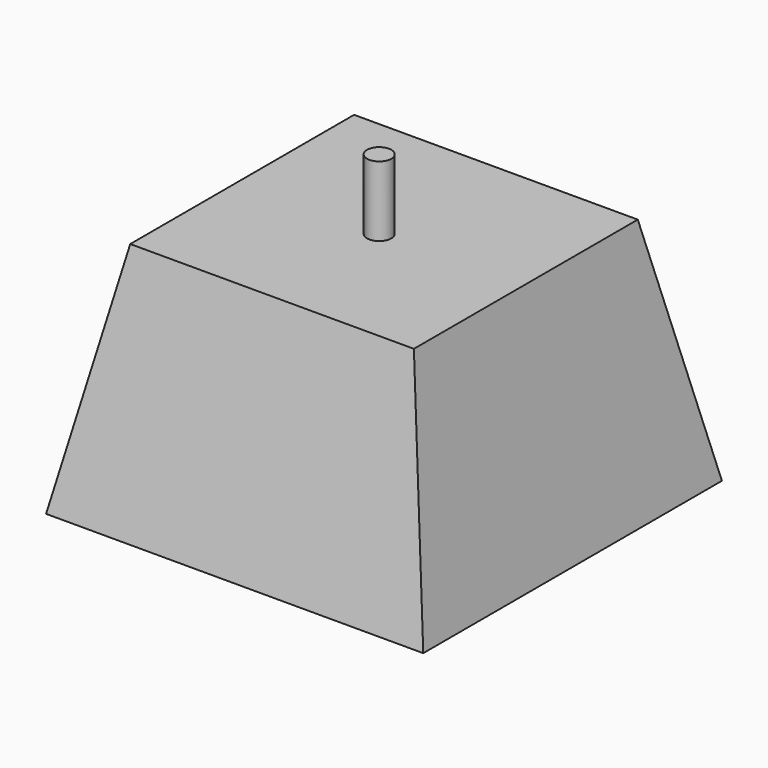
from build123d import *

# Parameters (mm, degrees)
F0_W     = 80.6774497032
F0_H     = 79.8543840647
F1_DEPTH = 50
F2_SIZE2 = 9.99999
F2_SIZE  = 49.99999
F3_R     = 2.5976453029
F4_DEPTH = 15


# Not quite as in the source:
# - a fillet or chamfer is up to 0.001 mm smaller than in the source, because OpenCascade refuses the exact size


with BuildPart() as f1:
    # F0 (on Top) → F1 (new body)
    with BuildSketch(Plane.XY):
        with Locations((0.1392643899, 1.1030137539)):
            Rectangle(F0_W, F0_H)
    extrude(amount=-F1_DEPTH)

    # F2 (size 50 and 10 in the source; OpenCascade refuses exactly that, so slightly less here)
    f2_edges = [f1.edges().sort_by_distance(p)[0] for p in [
        (0.139264, 41.030206, 0),
        (-40.19946, 1.103014, 0),
        (0.139264, -38.824178, 0),
        (40.477989, 1.103014, 0),
    ]]
    chamfer(f2_edges, length=F2_SIZE, length2=F2_SIZE2)

    # F3 (on Top) → F4 (join)
    with BuildSketch(Plane.XY):
        Circle(F3_R)
    extrude(amount=F4_DEPTH)


solid = f1.part
